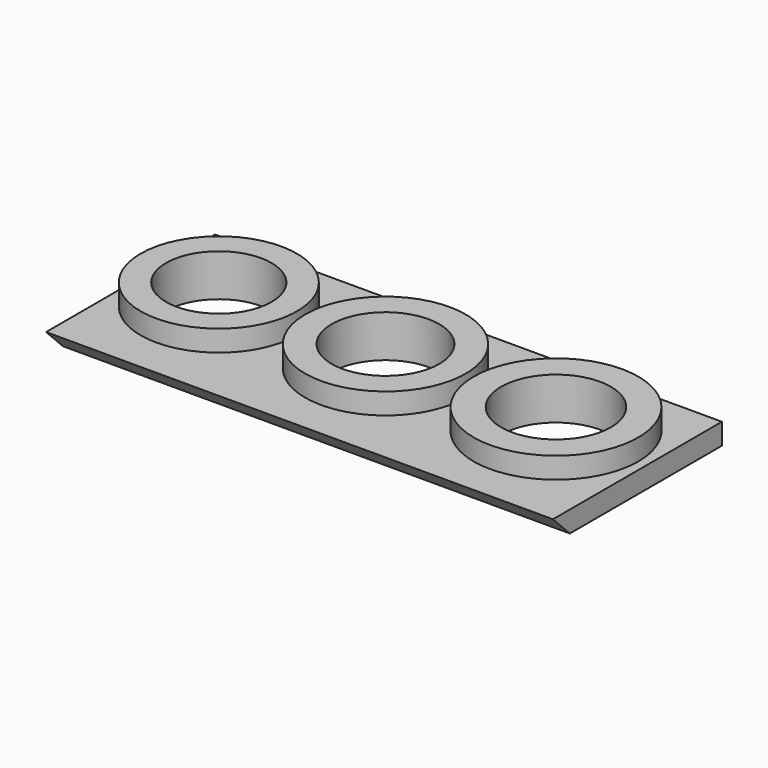
from build123d import *

# Parameters (mm, degrees)
F1_DEPTH = 2
F2_DEPTH = 1
F3_SIZE  = 0.99999


# Not quite as in the source:
# - a fillet or chamfer is up to 0.001 mm smaller than in the source, because OpenCascade refuses the exact size


with BuildPart() as f1:
    # F0 (on Top) → F1 (new body)
    with BuildSketch(Plane.XY):
        with BuildLine():
            ThreePointArc((-16.7408706831, 2.6987831955), (-20.4408706831, 6.3987831955), (-24.1408706831, 2.6987831955))
            Line((-24.1408706831, 2.6987831955), (-22.9408706831, 2.6987831955))
            ThreePointArc((-22.9408706831, 2.6987831955), (-20.4408706831, 5.1987831955), (-17.9408706831, 2.6987831955))
            Line((-17.9408706831, 2.6987831955), (-16.7408706831, 2.6987831955))
        make_face()
        with BuildLine():
            Line((-22.9408706831, 2.6987831955), (-24.1408706831, 2.6987831955))
            ThreePointArc((-24.1408706831, 2.6987831955), (-20.4408706831, -1.0012168045), (-16.7408706831, 2.6987831955))
            Line((-16.7408706831, 2.6987831955), (-17.9408706831, 2.6987831955))
            ThreePointArc((-17.9408706831, 2.6987831955), (-20.4408706831, 0.1987831955), (-22.9408706831, 2.6987831955))
        make_face()
    extrude(amount=F1_DEPTH)


with BuildPart() as f1b:
    # F0 (on Top) → F1, piece 2 (new body)
    with BuildSketch(Plane.XY):
        with BuildLine():
            ThreePointArc((-8.7494403885, 2.6987831955), (-12.5494403885, 6.4987831955), (-16.3494403885, 2.6987831955))
            Line((-16.3494403885, 2.6987831955), (-15.0994403885, 2.6987831955))
            ThreePointArc((-15.0994403885, 2.6987831955), (-12.5494403885, 5.2487831955), (-9.9994403885, 2.6987831955))
            Line((-9.9994403885, 2.6987831955), (-8.7494403885, 2.6987831955))
        make_face()
        with BuildLine():
            Line((-15.0994403885, 2.6987831955), (-16.3494403885, 2.6987831955))
            ThreePointArc((-16.3494403885, 2.6987831955), (-12.5494403885, -1.1012168045), (-8.7494403885, 2.6987831955))
            Line((-8.7494403885, 2.6987831955), (-9.9994403885, 2.6987831955))
            ThreePointArc((-9.9994403885, 2.6987831955), (-12.5494403885, 0.1487831955), (-15.0994403885, 2.6987831955))
        make_face()
    extrude(amount=F1_DEPTH)


with BuildPart() as f1c:
    # F0 (on Top) → F1, piece 3 (new body)
    with BuildSketch(Plane.XY):
        with BuildLine():
            Line((-1.874870298, 2.6987831955), (-0.574870298, 2.6987831955))
            ThreePointArc((-0.574870298, 2.6987831955), (-4.474870298, 6.5987831955), (-8.374870298, 2.6987831955))
            Line((-8.374870298, 2.6987831955), (-7.074870298, 2.6987831955))
            ThreePointArc((-7.074870298, 2.6987831955), (-4.474870298, 5.2987831955), (-1.874870298, 2.6987831955))
        make_face()
        with BuildLine():
            ThreePointArc((-8.374870298, 2.6987831955), (-4.474870298, -1.2012168045), (-0.574870298, 2.6987831955))
            Line((-0.574870298, 2.6987831955), (-1.874870298, 2.6987831955))
            ThreePointArc((-1.874870298, 2.6987831955), (-4.474870298, 0.0987831955), (-7.074870298, 2.6987831955))
            Line((-7.074870298, 2.6987831955), (-8.374870298, 2.6987831955))
        make_face()
    extrude(amount=F1_DEPTH)


with BuildPart() as f2:
    # F0 (on Top) → F2 (new body)
    with BuildSketch(Plane.XY):
        with BuildLine():
            Line((-0.1485164072, 7.1107540186), (-24.1485164072, 7.1107540186))
            Line((-24.1485164072, 7.1107540186), (-24.1485164072, 2.6987831955))
            Line((-24.1485164072, 2.6987831955), (-24.1408706831, 2.6987831955))
            ThreePointArc((-24.1408706831, 2.6987831955), (-20.4408706831, 6.3987831955), (-16.7408706831, 2.6987831955))
            Line((-16.7408706831, 2.6987831955), (-16.3494403885, 2.6987831955))
            ThreePointArc((-16.3494403885, 2.6987831955), (-12.5494403885, 6.4987831955), (-8.7494403885, 2.6987831955))
            Line((-8.7494403885, 2.6987831955), (-8.374870298, 2.6987831955))
            ThreePointArc((-8.374870298, 2.6987831955), (-4.474870298, 6.5987831955), (-0.574870298, 2.6987831955))
            Line((-0.574870298, 2.6987831955), (-0.1485164072, 2.6987831955))
            Line((-0.1485164072, 2.6987831955), (-0.1485164072, 7.1107540186))
        make_face()
        with BuildLine():
            Line((-24.1408706831, 2.6987831955), (-24.1485164072, 2.6987831955))
            Line((-24.1485164072, 2.6987831955), (-24.1485164072, -2.8892459814))
            Line((-24.1485164072, -2.8892459814), (-0.1485164072, -2.8892459814))
            Line((-0.1485164072, -2.8892459814), (-0.1485164072, 2.6987831955))
            Line((-0.1485164072, 2.6987831955), (-0.574870298, 2.6987831955))
            ThreePointArc((-0.574870298, 2.6987831955), (-4.474870298, -1.2012168045), (-8.374870298, 2.6987831955))
            Line((-8.374870298, 2.6987831955), (-8.7494403885, 2.6987831955))
            ThreePointArc((-8.7494403885, 2.6987831955), (-12.5494403885, -1.1012168045), (-16.3494403885, 2.6987831955))
            Line((-16.3494403885, 2.6987831955), (-16.7408706831, 2.6987831955))
            ThreePointArc((-16.7408706831, 2.6987831955), (-20.4408706831, -1.0012168045), (-24.1408706831, 2.6987831955))
        make_face()
    extrude(amount=F2_DEPTH)

    # F3 (size 1 in the source; OpenCascade refuses exactly that, so slightly less here)
    f3_edges = [f2.edges().sort_by_distance(p)[0] for p in [
        (-12.148516, -2.889246, 0),
    ]]
    chamfer(f3_edges, length=F3_SIZE)


solid = Compound([f1.part, f1b.part, f1c.part, f2.part])
